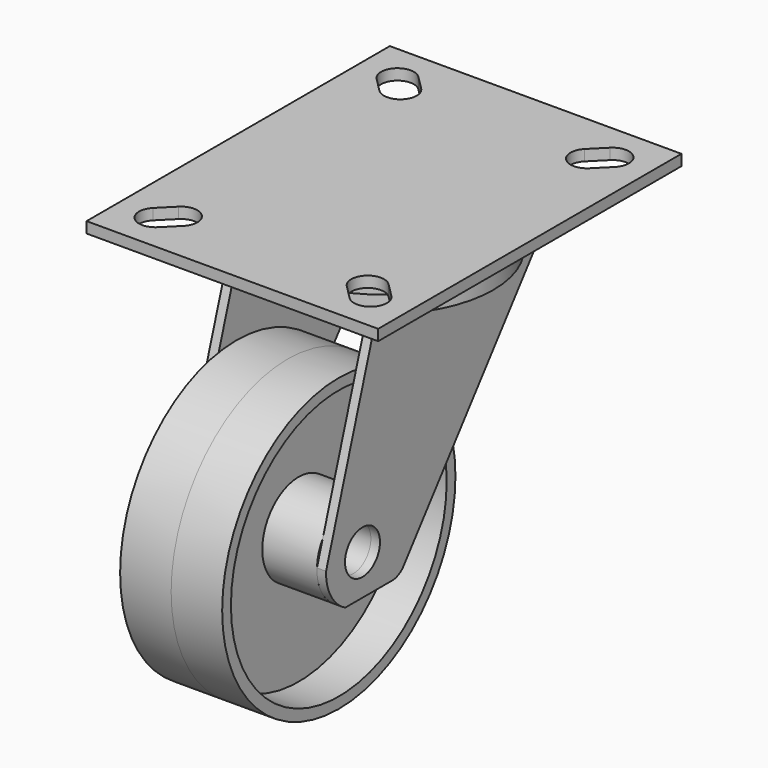
from build123d import *

# Parameters (mm, degrees)
F1_W      = 80
F1_H      = 104
F2_DEPTH  = 3
F3_R      = 40
F3_R_2    = 12.5
F4_DEPTH  = 14
F5_R      = 37
F5_R_2    = 12.5
F6_DEPTH  = 11
F3_R_3    = 6
F7_DEPTH  = 18
F9_R      = 32.5
F10_DEPTH = 6
F11_R     = 6
F12_DEPTH = 2.5
F14_R     = 30
F15_DEPTH = 6


with BuildPart() as f2:
    # F1 (on Top) → F2 (new body)
    with BuildSketch(Plane.XY):
        Rectangle(F1_W, F1_H)
        with BuildLine():
            Line((-32.6819805153, -38.3180194847), (-28.7928932188, -34.4289321881))
            ThreePointArc((-28.7928932188, -34.4289321881), (-22.4289321881, -34.4289321881), (-22.4289321881, -40.7928932188))
            Line((-22.4289321881, -40.7928932188), (-26.3180194847, -44.6819805153))
            ThreePointArc((-26.3180194847, -44.6819805153), (-32.6819805153, -44.6819805153), (-32.6819805153, -38.3180194847))
        make_face(mode=Mode.SUBTRACT)
        with BuildLine():
            ThreePointArc((32.6819805153, -38.3180194847), (32.6819805153, -44.6819805153), (26.3180194847, -44.6819805153))
            Line((26.3180194847, -44.6819805153), (22.4289321881, -40.7928932188))
            ThreePointArc((22.4289321881, -40.7928932188), (22.4289321881, -34.4289321881), (28.7928932188, -34.4289321881))
            Line((28.7928932188, -34.4289321881), (32.6819805153, -38.3180194847))
        make_face(mode=Mode.SUBTRACT)
        with BuildLine():
            ThreePointArc((-32.6819805153, 38.3180194847), (-32.6819805153, 44.6819805153), (-26.3180194847, 44.6819805153))
            Line((-26.3180194847, 44.6819805153), (-22.4289321881, 40.7928932188))
            ThreePointArc((-22.4289321881, 40.7928932188), (-22.4289321881, 34.4289321881), (-28.7928932188, 34.4289321881))
            Line((-28.7928932188, 34.4289321881), (-32.6819805153, 38.3180194847))
        make_face(mode=Mode.SUBTRACT)
        with BuildLine():
            Line((32.6819805153, 38.3180194847), (28.7928932188, 34.4289321881))
            ThreePointArc((28.7928932188, 34.4289321881), (22.4289321881, 34.4289321881), (22.4289321881, 40.7928932188))
            Line((22.4289321881, 40.7928932188), (26.3180194847, 44.6819805153))
            ThreePointArc((26.3180194847, 44.6819805153), (32.6819805153, 44.6819805153), (32.6819805153, 38.3180194847))
        make_face(mode=Mode.SUBTRACT)
    extrude(amount=-F2_DEPTH)

    # F9 (on face) → F10 (join)
    with BuildSketch(Plane(origin=(0, 0, -3), x_dir=(1, 0, 0), z_dir=(0, 0, -1))):
        Circle(F9_R)
    extrude(amount=F10_DEPTH)


with BuildPart() as f4:
    # F3 (on Right) → F4 (new body)
    with BuildSketch(Plane.YZ):
        with Locations((-33, -68)):
            Circle(F3_R)
        with Locations((-33, -68)):
            Circle(F3_R_2, mode=Mode.SUBTRACT)
    extrude(amount=F4_DEPTH)

    # F5 (on face) → F6 (cut)
    with BuildSketch(Plane.YZ.offset(14)):
        with Locations((-33, -68)):
            Circle(F5_R)
        with Locations((-33, -68)):
            Circle(F5_R_2, mode=Mode.SUBTRACT)
    extrude(amount=-F6_DEPTH, mode=Mode.SUBTRACT)

    # F3 (on Right) → F7 (join)
    with BuildSketch(Plane.YZ):
        with Locations((-33, -68)):
            Circle(F3_R_2)
        with Locations((-33, -68)):
            Circle(F3_R_3, mode=Mode.SUBTRACT)
    extrude(amount=F7_DEPTH)

    # F8: F4 across plane


with BuildPart() as f4_1:
    add(f4.part)
    add(f4.part.mirror(Plane.YZ))


with BuildPart() as f12:
    # F11 (on face) → F12 (new body)
    with BuildSketch(Plane.YZ.offset(18)):
        with BuildLine():
            ThreePointArc((-20.5, -68), (-22.266129945, -74.4057812672), (-27.0654453829, -79.0014117956))
            Line((-27.0654453829, -79.0014117956), (-22.8563387324, -79.0014117956))
            ThreePointArc((-22.8563387324, -79.0014117956), (-20.651853104, -78.4892000163), (-18.899032878, -77.0575090412))
            Line((-18.899032878, -77.0575090412), (27.8291888535, -16.5496617556))
            Line((27.8291888535, -16.5496617556), (27.8291888535, -13.9453392476))
            Line((27.8291888535, -13.9453392476), (-28.5524237418, -13.9453392476))
            Line((-28.5524237418, -13.9453392476), (-43.4908901592, -61.2035874413))
            ThreePointArc((-43.4908901592, -61.2035874413), (-29.4564232046, -56.0127958433), (-20.5, -68))
        make_face()
        with BuildLine():
            ThreePointArc((-45.4912247538, -67.5317007898), (-43.8519999998, -74.2035551101), (-38.9345546171, -79.0014117956))
            Line((-38.9345546171, -79.0014117956), (-27.0654453829, -79.0014117956))
            ThreePointArc((-27.0654453829, -79.0014117956), (-22.266129945, -74.4057812672), (-20.5, -68))
            ThreePointArc((-20.5, -68), (-29.4564232046, -56.0127958433), (-43.4908901592, -61.2035874413))
            Line((-43.4908901592, -61.2035874413), (-45.4912247538, -67.5317007898))
        make_face()
        with Locations((-33, -68)):
            Circle(F11_R, mode=Mode.SUBTRACT)
    extrude(amount=F12_DEPTH)


with BuildPart() as f13_1:
    # F13: instance of F12
    add(f12.part.mirror(Plane.YZ))


with BuildPart() as f12_1:
    add(f12.part)

    add(f13_1.part)  # F15 merges F13_1
    # F14 (on face) → F15 (join)
    with BuildSketch(Plane(origin=(0, 0, -9), x_dir=(1, 0, 0), z_dir=(0, 0, -1))):
        Circle(F14_R)
    extrude(amount=F15_DEPTH)


solid = Compound([f2.part, f4_1.part, f12_1.part])
